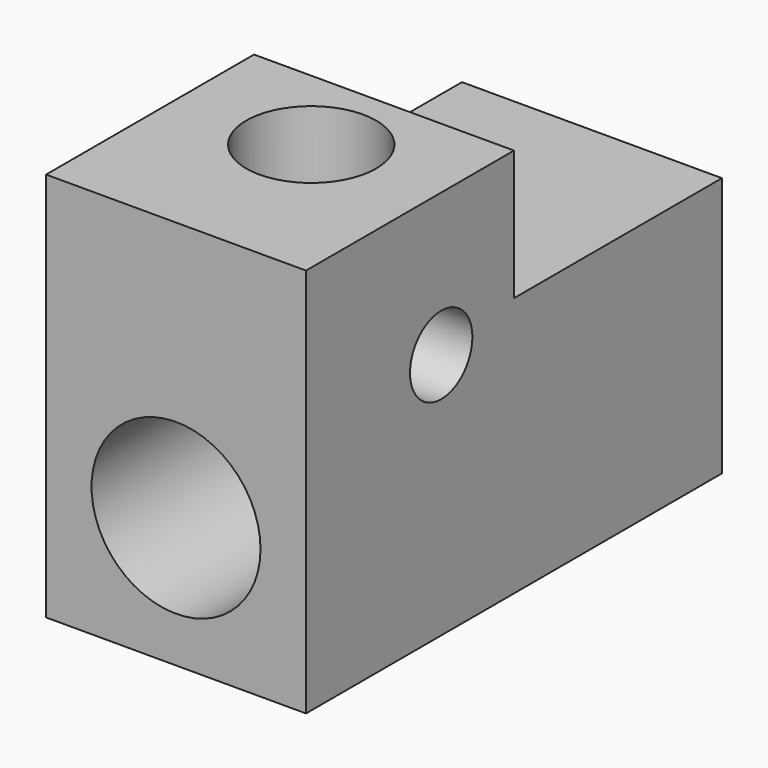
from build123d import *

# Parameters (mm, degrees)
F0_W          = 10
F0_H          = 10
F0_R          = 3.25
F1_DEPTH      = 10
F0_H_2        = 5
F2_DEPTH      = 10
F3_R          = 4.25
F3_R_2        = 3.25
F4_DEPTH      = 10
F5_R          = 1.5
F6_DEPTH      = 5.001
F6_DEPTH_BACK = 5.001
F7_R          = 2.5
F8_DEPTH      = 10


with BuildPart() as f1:
    # F0 (on Front) → F1 (new body)
    with BuildSketch(Plane.XZ):
        Rectangle(F0_W, F0_H)
        Circle(F0_R, mode=Mode.SUBTRACT)
    extrude(amount=-F1_DEPTH)

    # F0 (on Front) → F2 (join)
    with BuildSketch(Plane.XZ):
        with Locations((0, 7.5)):
            Rectangle(F0_W, F0_H_2)
        Rectangle(F0_W, F0_H)
        Circle(F0_R, mode=Mode.SUBTRACT)
    extrude(amount=F2_DEPTH)

    # F3 (on face) → F4 (cut)
    with BuildSketch(Plane(origin=(0, 10, 0), x_dir=(-1, 0, 0), z_dir=(0, 1, 0))):
        Circle(F3_R)
        Circle(F3_R_2, mode=Mode.SUBTRACT)
        Circle(F3_R_2)
    extrude(amount=-F4_DEPTH, mode=Mode.SUBTRACT)

    # F5 (on Right) → F6 (cut, two sides)
    with BuildSketch(Plane.YZ) as f6_sk:
        with Locations((-3.5, 4.5)):
            Circle(F5_R)
    extrude(amount=-F6_DEPTH, mode=Mode.SUBTRACT)
    extrude(f6_sk.sketch, amount=F6_DEPTH_BACK, mode=Mode.SUBTRACT)

    # F7 (on face) → F8 (cut)
    with BuildSketch(Plane.XY.offset(10)):
        with Locations((0, -3.5)):
            Circle(F7_R)
    extrude(amount=-F8_DEPTH, mode=Mode.SUBTRACT)


solid = f1.part
